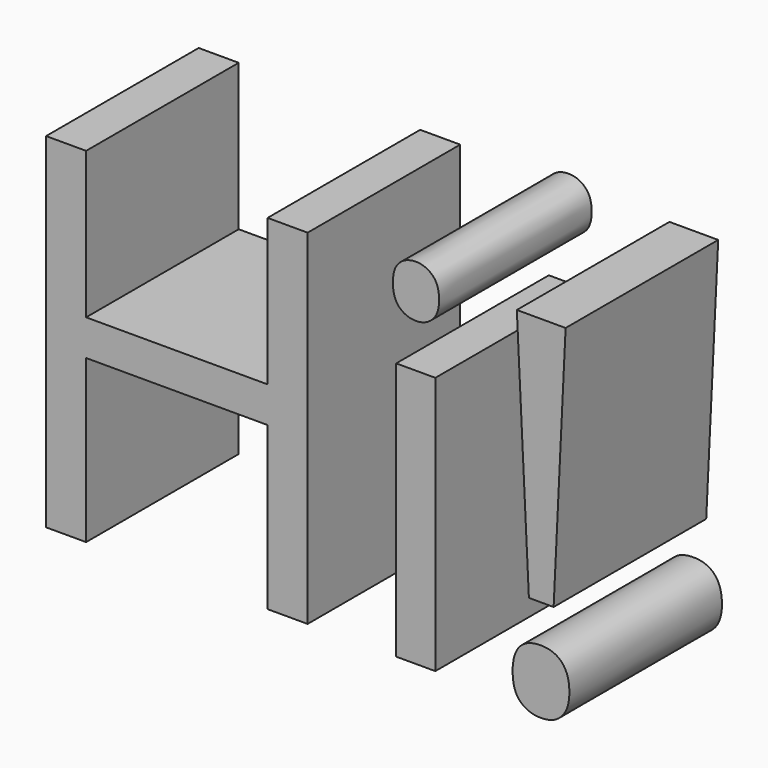
from build123d import *

# Parameters (mm, degrees)
F0_TEXT_SIZE = 192.761566076
F1_DEPTH     = 76.2


# Not quite as in the source:
# - Text() gives the source's letters only with a copy of the font that has no kerning and outlines rounded to 1/6400 em; it was checked with that copy


with BuildPart() as f1:
    # F0 (on Front) → F1 (new body)
    with BuildSketch(Plane.XZ):
        with Locations((-71.9643086195, -64.5394250751)):
            Text('Hi!', F0_TEXT_SIZE, font='Open Sans', text_align=(TextAlign.LEFT, TextAlign.BOTTOM))
    extrude(amount=F1_DEPTH)


solid = f1.part
